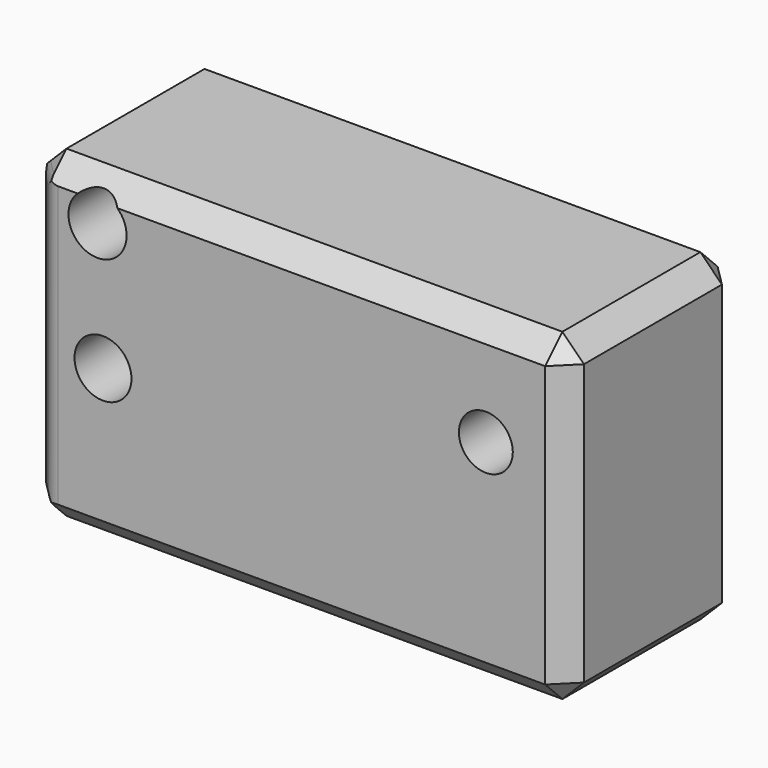
from build123d import *

# Parameters (mm, degrees)
F0_W         = 127
F0_H         = 76.2
F0_R         = 6.8502620854
F0_R_2       = 6.35
F1_DEPTH     = 50.8
F2_R         = 6.7087058048
F3_DEPTH     = 127
F4_T1_DEPTH  = 6.4524666085
F4_T3_DEPTH  = 6.4524666085
F4_T5_DEPTH  = 6.4524666085
F4_T7_DEPTH  = 6.4524666085
F4_T9_DEPTH  = 6.4524666085
F4_T11_DEPTH = 6.4524666085
F4_T13_DEPTH = 6.4524666085
F4_T15_DEPTH = 6.4524666085
F4_T17_DEPTH = 102.3282991577
F4_T19_DEPTH = 153.1282991577
F4_T21_DEPTH = 76.9282991577
F5_T1_DEPTH  = 15.2572709249
F5_T3_DEPTH  = 76.5610244843


# Not quite as in the source:
# - a fillet or chamfer that OpenCascade refuses, or shapes differently, is made with other operations: its cross-section is extruded or revolved along the edge and cut away or added


with BuildPart() as f1:
    # F0 (on Front) → F1 (new body)
    with BuildSketch(Plane.XZ):
        with Locations((-63.5, 38.1)):
            Rectangle(F0_W, F0_H)
        with Locations((-110.5553433299, 66.1175847054)):
            Circle(F0_R, mode=Mode.SUBTRACT)
        with Locations((-19.05, 50.8)):
            Circle(F0_R_2, mode=Mode.SUBTRACT)
    extrude(amount=F1_DEPTH)

    # F2 (on face) → F3 (cut)
    with BuildSketch(Plane.XZ.offset(50.8)):
        with Locations((-109.2690080404, 36.7891639471)):
            Circle(F2_R)
    extrude(amount=-F3_DEPTH, mode=Mode.SUBTRACT)

    # F4: chamfer of 5.08 on 12 edges, made by hand

    # F4_s2 → F4_t1 (cut)
    with BuildSketch(Plane(origin=(-81.28, -81.28, 81.28), x_dir=(0.7071067812, -0.7071067812, 0), z_dir=(-0.5773502692, -0.5773502692, 0.5773502692))):
        Polygon((-53.8815367264, -6.2217039467), (-57.4736391748, -12.4434078933), (-50.289434278, -12.4434078933), align=None)
    extrude(amount=F4_T1_DEPTH, mode=Mode.SUBTRACT)

    # F4_s4 → F4_t3 (cut)
    with BuildSketch(Plane(origin=(-55.88, -55.88, -55.88), x_dir=(0.7071067812, -0.7071067812, 0), z_dir=(-0.5773502692, -0.5773502692, -0.5773502692))):
        Polygon((-57.4736391748, 74.66044736), (-50.289434278, 74.66044736), (-53.8815367264, 68.4387434134), align=None)
    extrude(amount=F4_T3_DEPTH, mode=Mode.SUBTRACT)

    # F4_s6 → F4_t5 (cut)
    with BuildSketch(Plane(origin=(38.9466666667, -38.9466666667, 38.9466666667), x_dir=(0.7071067812, 0.7071067812, 0), z_dir=(0.5773502692, -0.5773502692, 0.5773502692))):
        Polygon((-35.9210244843, 45.6258289422), (-32.3289220358, 39.4041249956), (-39.5131269327, 39.4041249956), align=None)
    extrude(amount=F4_T5_DEPTH, mode=Mode.SUBTRACT)

    # F4_s8 → F4_t7 (cut)
    with BuildSketch(Plane(origin=(-64.3466666667, 64.3466666667, 64.3466666667), x_dir=(-0.7071067812, -0.7071067812, 0), z_dir=(-0.5773502692, 0.5773502692, 0.5773502692))):
        Polygon((89.8025612107, 14.5173092089), (93.3946636591, 8.2956052622), (86.2104587623, 8.2956052622), align=None)
    extrude(amount=F4_T7_DEPTH, mode=Mode.SUBTRACT)

    # F4_s10 → F4_t9 (cut)
    with BuildSketch(Plane(origin=(-38.9466666667, 38.9466666667, -38.9466666667), x_dir=(-0.7071067812, -0.7071067812, 0), z_dir=(-0.5773502692, 0.5773502692, -0.5773502692))):
        Polygon((93.3946636591, 53.9214342045), (86.2104587623, 53.9214342045), (89.8025612107, 47.6997302578), align=None)
    extrude(amount=F4_T9_DEPTH, mode=Mode.SUBTRACT)

    # F4_s12 → F4_t11 (cut)
    with BuildSketch(Plane(origin=(22.0133333333, 22.0133333333, 22.0133333333), x_dir=(-0.7071067812, 0.7071067812, 0), z_dir=(0.5773502692, 0.5773502692, 0.5773502692))):
        Polygon((0, 66.3648420978), (-3.5921024484, 60.1431381511), (3.5921024484, 60.1431381511), align=None)
    extrude(amount=F4_T11_DEPTH, mode=Mode.SUBTRACT)

    # F4_s14 → F4_t13 (cut)
    with BuildSketch(Plane(origin=(-3.3866666667, -3.3866666667, 3.3866666667), x_dir=(-0.7071067812, 0.7071067812, 0), z_dir=(0.5773502692, 0.5773502692, -0.5773502692))):
        Polygon((-3.5921024484, 2.0739013156), (3.5921024484, 2.0739013156), (0, -4.1478026311), align=None)
    extrude(amount=F4_T13_DEPTH, mode=Mode.SUBTRACT)

    # F4_s16 → F4_t15 (cut)
    with BuildSketch(Plane(origin=(13.5466666667, -13.5466666667, -13.5466666667), x_dir=(0.7071067812, 0.7071067812, 0), z_dir=(0.5773502692, -0.5773502692, -0.5773502692))):
        Polygon((-32.3289220358, 22.8129144711), (-39.5131269327, 22.8129144711), (-35.9210244843, 16.5912105245), align=None)
    extrude(amount=F4_T15_DEPTH, mode=Mode.SUBTRACT)

    # F4_s18 → F4_t17 (cut)
    with BuildSketch(Plane.XY.offset(-13.0641495789)):
        Polygon((-127, -45.72), (-121.92, -50.8), (-127, -50.8), align=None)
        Polygon((-127, -5.08), (-121.92, 0), (-127, 0), align=None)
        Polygon((0, -45.72), (-5.08, -50.8), (0, -50.8), align=None)
        Polygon((0, -5.08), (-5.08, 0), (0, 0), align=None)
    extrude(amount=F4_T17_DEPTH, mode=Mode.SUBTRACT)

    # F4_s20 → F4_t19 (cut)
    with BuildSketch(Plane.YZ.offset(-140.0641495789)):
        Polygon((-45.72, 76.2), (-50.8, 71.12), (-50.8, 76.2), align=None)
        Polygon((-5.08, 76.2), (0, 71.12), (0, 76.2), align=None)
        Polygon((0, 5.08), (-5.08, 0), (0, 0), align=None)
        Polygon((-50.8, 5.08), (-45.72, 0), (-50.8, 0), align=None)
    extrude(amount=F4_T19_DEPTH, mode=Mode.SUBTRACT)

    # F4_s22 → F4_t21 (cut)
    with BuildSketch(Plane.XZ.offset(-13.0641495789)):
        Polygon((-127, 5.08), (-121.92, 0), (-127, 0), align=None)
        Polygon((-121.92, 76.2), (-127, 71.12), (-127, 76.2), align=None)
        Polygon((0, 5.08), (-5.08, 0), (0, 0), align=None)
        Polygon((-5.08, 76.2), (0, 71.12), (0, 76.2), align=None)
    extrude(amount=F4_T21_DEPTH, mode=Mode.SUBTRACT)

    # F5: fillet of radius 5.08 on 4 edges, made by hand

    # F5_s2 → F5_t1 (cut)
    with BuildSketch(Plane(origin=(-43.4942598667, 43.4942598667, 0), x_dir=(0, 0, 1), z_dir=(0.7071067812, -0.7071067812, 0))):
        with BuildLine():
            ThreePointArc((6.6946132056, 122.1314832465), (5.1558535372, 121.892827965), (3.7616738381, 121.1992858777))
            Line((3.7616738381, 121.1992858777), (5.08, 122.1314832465))
            Line((5.08, 122.1314832465), (6.6946132056, 122.1314832465))
        make_face()
        with BuildLine():
            ThreePointArc((72.4383261619, 121.1992858777), (71.0441464628, 121.892827965), (69.5053867944, 122.1314832465))
            Line((69.5053867944, 122.1314832465), (71.12, 122.1314832465))
            Line((71.12, 122.1314832465), (72.4383261619, 121.1992858777))
        make_face()
    extrude(amount=F5_T1_DEPTH, mode=Mode.SUBTRACT)

    # F5_s4 → F5_t3 (cut)
    with BuildSketch(Plane.XY.offset(-0.1805122422)):
        with BuildLine():
            ThreePointArc((-119.8157951031, -50.8), (-121.7598269396, -50.4133080252), (-123.4078975516, -49.3121024484))
            Line((-123.4078975516, -49.3121024484), (-121.92, -50.8))
            Line((-121.92, -50.8), (-119.8157951031, -50.8))
        make_face()
        with BuildLine():
            ThreePointArc((-127, -43.6157951031), (-126.6133080252, -45.5598269396), (-125.5121024484, -47.2078975516))
            Line((-125.5121024484, -47.2078975516), (-127, -45.72))
            Line((-127, -45.72), (-127, -43.6157951031))
        make_face()
    extrude(amount=F5_T3_DEPTH, mode=Mode.SUBTRACT)


solid = f1.part
